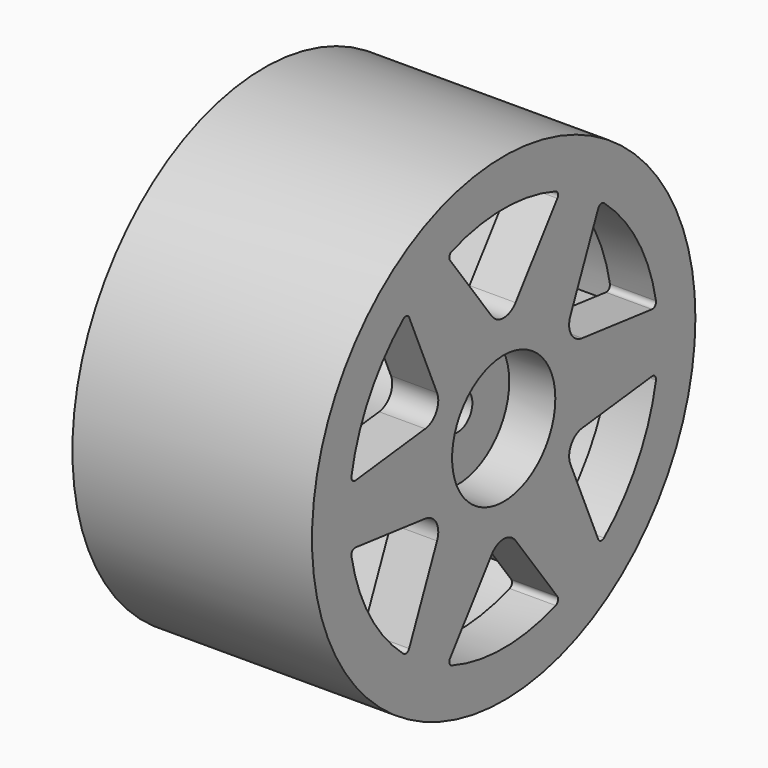
from build123d import *
from build123d import SkipClean  # not in build123d's __all__

# Parameters (mm, degrees)
F0_R      = 26
F1_DEPTH  = 26
F3_R      = 23.15
F4_DEPTH  = 21
F5_R      = 8.7
F6_DEPTH  = 12.5
F8_DEPTH  = 25
F9_R      = 7
F10_DEPTH = 5
F11_R     = 2
F12_DEPTH = 25
F13_W     = 5
F13_H     = 4.1104049385
F16_DEPTH = 25
F19_R     = 2
F20_R     = 0.5


with BuildPart() as f1:
    # F0 (on Right) → F1 (new body)
    with BuildSketch(Plane.YZ):
        Circle(F0_R)
    extrude(amount=F1_DEPTH)

    # F3 (on Right) → F4 (cut)
    with BuildSketch(Plane.YZ):
        Circle(F3_R)
    extrude(amount=F4_DEPTH, mode=Mode.SUBTRACT)

    # F5 (on offset) → F6 (join)
    with BuildSketch(Plane.YZ.offset(26)):
        Circle(F5_R)
    extrude(amount=-F6_DEPTH)

    # F7 (on offset) → F8 (cut)
    with BuildSketch(Plane.YZ.offset(26)):
        Polygon((-22.9713798889, 2.8702275171), (-7.9674337148, 4.6), (-13.9713798889, 18.4586847852), align=None)
        Polygon((-9, 21.3289123023), (0, 9.2), (9, 21.3289123023), align=None)
        Polygon((13.9713798889, 18.4586847852), (7.9674337148, 4.6), (22.9713798889, 2.8702275171), align=None)
        Polygon((22.9713798889, -2.8702275171), (7.9674337148, -4.6), (13.9713798889, -18.4586847852), align=None)
        Polygon((9, -21.3289123023), (0, -9.2), (-9, -21.3289123023), align=None)
        Polygon((-13.9713798889, -18.4586847852), (-7.9674337148, -4.6), (-22.9713798889, -2.8702275171), align=None)
    extrude(amount=-F8_DEPTH, mode=Mode.SUBTRACT)

    # F9 (on offset) → F10 (cut)
    with BuildSketch(Plane.YZ.offset(26)):
        Circle(F9_R)
    extrude(amount=-F10_DEPTH, mode=Mode.SUBTRACT)

    # F11 (on offset) → F12 (cut)
    with BuildSketch(Plane.YZ.offset(26)):
        Circle(F11_R)
    extrude(amount=-F12_DEPTH, mode=Mode.SUBTRACT)

    # F13 (on Front) → F14 (revolve)
    with BuildSketch(Plane.XZ):
        with Locations((23.5, 23.0552024692)):
            Rectangle(F13_W, F13_H)
    revolve(axis=Axis((13.1547623314, 0, 0), (1, 0, 0)))

    # F15 (on Right) → F16 (join)
    with BuildSketch(Plane.YZ):
        Polygon((12.9330127019, 21.4006350946), (12.5, 21.6506350946), (12.0669872981, 21.9006350946), (3.5669872981, 7.1782032303), (4.4330127019, 6.6782032303), align=None)
        Polygon((-3.5669872981, 7.1782032303), (-12.0669872981, 21.9006350946), (-12.5, 21.6506350946), (-12.9330127019, 21.4006350946), (-4.4330127019, 6.6782032303), align=None)
        Polygon((-8, 0.5), (-25, 0.5), (-25, 0), (-25, -0.5), (-8, -0.5), align=None)
        Polygon((-4.4330127019, -6.6782032303), (-12.9330127019, -21.4006350946), (-12.5, -21.6506350946), (-12.0669872981, -21.9006350946), (-3.5669872981, -7.1782032303), align=None)
        Polygon((3.5669872981, -7.1782032303), (12.0669872981, -21.9006350946), (12.5, -21.6506350946), (12.9330127019, -21.4006350946), (4.4330127019, -6.6782032303), align=None)
        Polygon((8, -0.5), (25, -0.5), (25, 0), (25, 0.5), (8, 0.5), align=None)
    extrude(amount=F16_DEPTH)

    # F17 (on Front) → F18 (revolve, cut)
    with BuildSketch(Plane.XZ):
        Polygon((14.5, 23.15), (-3.0704529053, 23.15), (-1.8057800443, 5.6787895144), (13.5, 5.6787895144), (13.5, 8.7), (14.5, 8.7), align=None)
    with SkipClean():  # cleaning this boolean's faces spoils the solid; the shape is the same uncleaned
        revolve(axis=Axis((9.9325310439, 0, 0), (1, 0, 0)), mode=Mode.SUBTRACT)

    # F19
    f19_edges = [f1.edges().sort_by_distance(p)[0] for p in [
        (23.5, -7.967434, 4.6),
        (23.5, 0, 9.2),
        (23.5, 7.967434, 4.6),
        (23.5, 7.967434, -4.6),
        (23.5, 0, -9.2),
        (23.5, -7.967434, -4.6),
    ]]
    fillet(f19_edges, radius=F19_R)

    # F20
    f20_edges = [f1.edges().sort_by_distance(p)[0] for p in [
        (23.5, 20.766266, -3.12445),
        (23.5, 13.088986, -16.421889),
        (23.5, 20.766266, 3.12445),
        (23.5, 13.088986, 16.421889),
        (23.5, 7.67728, -19.546339),
        (23.5, 7.67728, 19.546339),
        (23.5, -7.67728, 19.546339),
        (23.5, -13.088986, 16.421889),
        (23.5, -20.766266, 3.12445),
        (23.5, -20.766266, -3.12445),
        (23.5, -13.088986, -16.421889),
        (23.5, -7.67728, -19.546339),
    ]]
    fillet(f20_edges, radius=F20_R)


solid = f1.part
